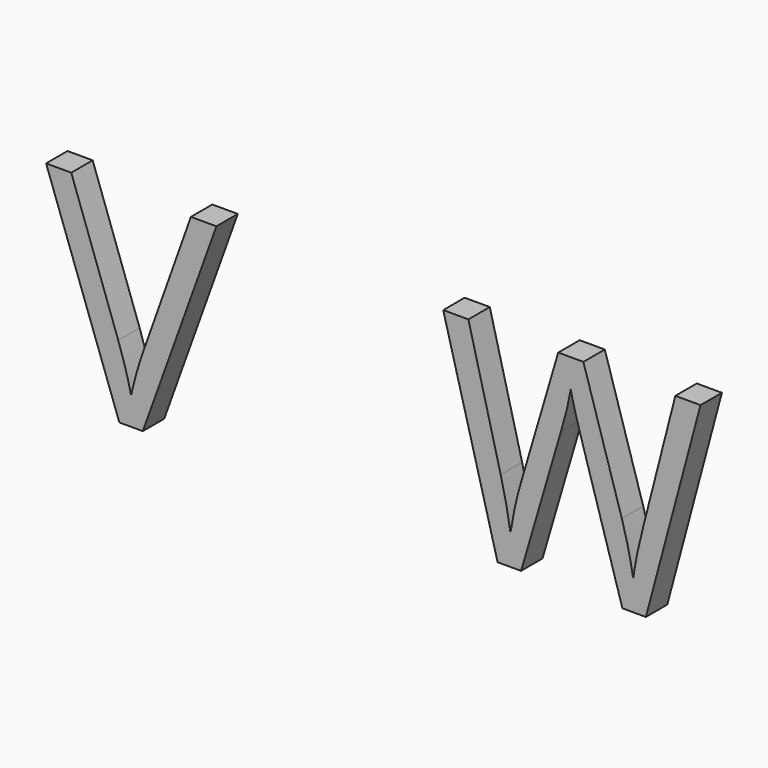
from build123d import *

# Parameters (mm, degrees)
F0_TEXT_SIZE = 135.7550577571
F1_DEPTH     = 12.7


# Not quite as in the source:
# - Text() gives the source's letters only with a copy of the font that has no kerning and outlines rounded to 1/6400 em; it was checked with that copy


with BuildPart() as f1:
    # F0 (on Front) → F1 (new body)
    with BuildSketch(Plane.XZ):
        with Locations((-57.4111714959, -56.2400110066)):
            Text('V   W', F0_TEXT_SIZE, font='Open Sans', text_align=(TextAlign.LEFT, TextAlign.BOTTOM))
    extrude(amount=F1_DEPTH)


solid = f1.part
